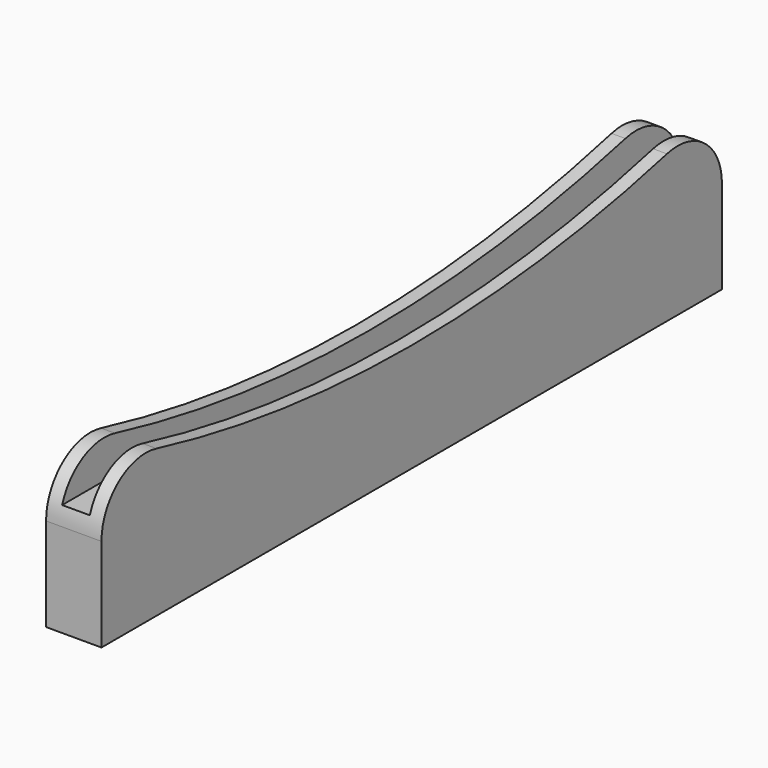
from build123d import *

# Parameters (mm, degrees)
F0_W        = 152.4
F0_H        = 3.175
F1_DEPTH    = 6.35
F2_DEPTH    = 3.175
F3_T1_DEPTH = 86.5404436654
F3_T3_DEPTH = 86.5404436654


# Not quite as in the source:
# - a fillet or chamfer that OpenCascade refuses, or shapes differently, is made with other operations: its cross-section is extruded or revolved along the edge and cut away or added


with BuildPart() as f1:
    # F0 (on Right) → F1 (new body, symmetric)
    with BuildSketch(Plane.YZ):
        with Locations((88.9, 1.5875)):
            Rectangle(F0_W, F0_H)
        Polygon((0, 25.4), (0, 0), (12.7, 0), (12.7, 3.175), (12.7, 25.4), align=None)
        Polygon((165.1, 3.175), (165.1, 0), (177.8, 0), (177.8, 25.4), (165.1, 25.4), align=None)
        with BuildLine():
            Line((0, 38.1), (0, 25.4))
            Line((0, 25.4), (12.7, 25.4))
            Line((12.7, 25.4), (12.7, 3.175))
            Line((12.7, 3.175), (165.1, 3.175))
            Line((165.1, 3.175), (165.1, 25.4))
            Line((165.1, 25.4), (177.8, 25.4))
            Line((177.8, 25.4), (177.8, 38.1))
            ThreePointArc((177.8, 38.1), (88.9, 24.8473031945), (0, 38.1))
        make_face()
    extrude(amount=F1_DEPTH, both=True)

    # F0 (on Right) → F2 (cut, symmetric)
    with BuildSketch(Plane.YZ):
        with BuildLine():
            Line((0, 38.1), (0, 25.4))
            Line((0, 25.4), (12.7, 25.4))
            Line((12.7, 25.4), (12.7, 3.175))
            Line((12.7, 3.175), (165.1, 3.175))
            Line((165.1, 3.175), (165.1, 25.4))
            Line((165.1, 25.4), (177.8, 25.4))
            Line((177.8, 25.4), (177.8, 38.1))
            ThreePointArc((177.8, 38.1), (88.9, 24.8473031945), (0, 38.1))
        make_face()
    extrude(amount=F2_DEPTH, both=True, mode=Mode.SUBTRACT)

    # F3: fillet of radius 12.7 on 4 edges, made by hand

    # F3_s2 → F3_t1 (cut)
    with BuildSketch(Plane.YZ.offset(-48.0327218327)):
        with BuildLine():
            ThreePointArc((0, 21.4269112669), (4.8711942162, 31.4269012669), (15.748, 33.755726944))
            ThreePointArc((15.748, 33.755726944), (7.8448900248, 35.8223397437), (0, 38.1))
            Line((0, 38.1), (0, 21.4269112669))
        make_face()
        with BuildLine():
            ThreePointArc((177.8, 21.4269112669), (172.9288057838, 31.4269012669), (162.052, 33.755726944))
            ThreePointArc((162.052, 33.755726944), (169.9551099752, 35.8223397437), (177.8, 38.1))
            Line((177.8, 38.1), (177.8, 21.4269112669))
        make_face()
    extrude(amount=F3_T1_DEPTH, mode=Mode.SUBTRACT)

    # F3_s4 → F3_t3 (cut)
    with BuildSketch(Plane.YZ.offset(-38.5077218327)):
        with BuildLine():
            ThreePointArc((0, 21.4269112669), (4.8711942162, 31.4269012669), (15.748, 33.755726944))
            ThreePointArc((15.748, 33.755726944), (7.8448900248, 35.8223397437), (0, 38.1))
            Line((0, 38.1), (0, 21.4269112669))
        make_face()
        with BuildLine():
            ThreePointArc((177.8, 21.4269112669), (172.9288057838, 31.4269012669), (162.052, 33.755726944))
            ThreePointArc((162.052, 33.755726944), (169.9551099752, 35.8223397437), (177.8, 38.1))
            Line((177.8, 38.1), (177.8, 21.4269112669))
        make_face()
    extrude(amount=F3_T3_DEPTH, mode=Mode.SUBTRACT)


solid = f1.part
